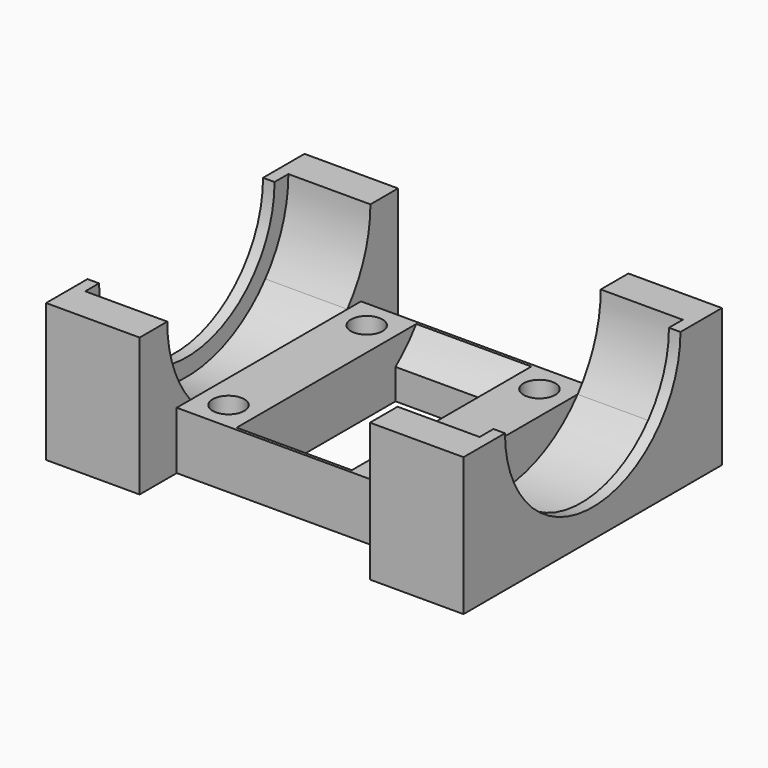
from build123d import *

# Parameters (mm, degrees)
F0_W      = 20
F0_H      = 20
F0_R      = 1.375
F0_W_2    = 10
F0_H_2    = 15
F1_DEPTH  = 5
F3_DEPTH  = 7.125
F6_DEPTH  = 7.125
F8_DEPTH  = 1
F10_DEPTH = 1
F11_R     = 12
F12_DEPTH = 5


with BuildPart() as f1:
    # F0 (on Top) → F1 (new body)
    with BuildSketch(Plane.XY):
        with Locations((10, 10)):
            Rectangle(F0_W, F0_H)
        with Locations((2.5, 2.5)):
            Circle(F0_R, mode=Mode.SUBTRACT)
        with Locations((17.5, 2.5)):
            Circle(F0_R, mode=Mode.SUBTRACT)
        with Locations((2.5, 17.5)):
            Circle(F0_R, mode=Mode.SUBTRACT)
        with Locations((10, 10)):
            Rectangle(F0_W_2, F0_H_2, mode=Mode.SUBTRACT)
        with Locations((17.5, 17.5)):
            Circle(F0_R, mode=Mode.SUBTRACT)
    extrude(amount=F1_DEPTH)

    # F2 (on face) → F3 (join)
    with BuildSketch(Plane(origin=(0, 0, 0), x_dir=(0, -1, 0), z_dir=(-1, 0, 0))):
        with BuildLine():
            ThreePointArc((-18.5176654665, 5), (-20.379255435, 8.2822477738), (-21.025, 12))
            Line((-21.025, 12), (-24.025, 12))
            Line((-24.025, 12), (-24.025, 0))
            Line((-24.025, 0), (-20, 0))
            Line((-20, 0), (-20, 5))
            Line((-20, 5), (-18.5176654665, 5))
        make_face()
        with BuildLine():
            ThreePointArc((-1.4823345335, 5), (-10, 0.975), (-18.5176654665, 5))
            Line((-18.5176654665, 5), (-20, 5))
            Line((-20, 5), (-20, 0))
            Line((-20, 0), (0, 0))
            Line((0, 0), (0, 5))
            Line((0, 5), (-1.4823345335, 5))
        make_face()
        with BuildLine():
            ThreePointArc((1.025, 12), (0.379255435, 8.2822477738), (-1.4823345335, 5))
            Line((-1.4823345335, 5), (0, 5))
            Line((0, 5), (0, 0))
            Line((0, 0), (4.025, 0))
            Line((4.025, 0), (4.025, 12))
            Line((4.025, 12), (1.025, 12))
        make_face()
    extrude(amount=F3_DEPTH)

    # F5 (on face) → F6 (join)
    with BuildSketch(Plane.YZ.offset(20)):
        with BuildLine():
            Line((0, 5), (1.4823345335, 5))
            ThreePointArc((1.4823345335, 5), (-0.379255435, 8.2822477738), (-1.025, 12))
            Line((-1.025, 12), (-4.025, 12))
            Line((-4.025, 12), (-4.025, 0))
            Line((-4.025, 0), (0, 0))
            Line((0, 0), (0, 5))
        make_face()
        with BuildLine():
            ThreePointArc((18.5176654665, 5), (10, 0.975), (1.4823345335, 5))
            Line((1.4823345335, 5), (0, 5))
            Line((0, 5), (0, 0))
            Line((0, 0), (20, 0))
            Line((20, 0), (20, 5))
            Line((20, 5), (18.5176654665, 5))
        make_face()
        with BuildLine():
            ThreePointArc((21.025, 12), (20.379255435, 8.2822477738), (18.5176654665, 5))
            Line((18.5176654665, 5), (20, 5))
            Line((20, 5), (20, 0))
            Line((20, 0), (24.025, 0))
            Line((24.025, 0), (24.025, 12))
            Line((24.025, 12), (21.025, 12))
        make_face()
    extrude(amount=F6_DEPTH)

    # F7 (on face) → F8 (join)
    with BuildSketch(Plane.YZ.offset(27.125)):
        with BuildLine():
            Line((0.475, 12), (-1.025, 12))
            ThreePointArc((-1.025, 12), (10, 0.975), (21.025, 12))
            Line((21.025, 12), (19.525, 12))
            ThreePointArc((19.525, 12), (10, 2.475), (0.475, 12))
        make_face()
        with BuildLine():
            Line((-4.025, 12), (-4.025, 0))
            Line((-4.025, 0), (24.025, 0))
            Line((24.025, 0), (24.025, 12))
            Line((24.025, 12), (21.025, 12))
            ThreePointArc((21.025, 12), (10, 0.975), (-1.025, 12))
            Line((-1.025, 12), (-4.025, 12))
        make_face()
    extrude(amount=F8_DEPTH)

    # F9 (on face) → F10 (join)
    with BuildSketch(Plane(origin=(-7.125, 0, 0), x_dir=(0, -1, 0), z_dir=(-1, 0, 0))):
        with BuildLine():
            Line((-19.525, 12), (-21.025, 12))
            ThreePointArc((-21.025, 12), (-10, 0.975), (1.025, 12))
            Line((1.025, 12), (-0.475, 12))
            ThreePointArc((-0.475, 12), (-10, 2.475), (-19.525, 12))
        make_face()
        with BuildLine():
            Line((-21.025, 12), (-24.025, 12))
            Line((-24.025, 12), (-24.025, 0))
            Line((-24.025, 0), (4.025, 0))
            Line((4.025, 0), (4.025, 12))
            Line((4.025, 12), (1.025, 12))
            ThreePointArc((1.025, 12), (-10, 0.975), (-21.025, 12))
        make_face()
    extrude(amount=F10_DEPTH)

    # F11 (on offset) → F12 (cut, symmetric)
    with BuildSketch(Plane.YZ.offset(10)):
        with Locations((10, 12)):
            Circle(F11_R)
    extrude(amount=F12_DEPTH, both=True, mode=Mode.SUBTRACT)


solid = f1.part
